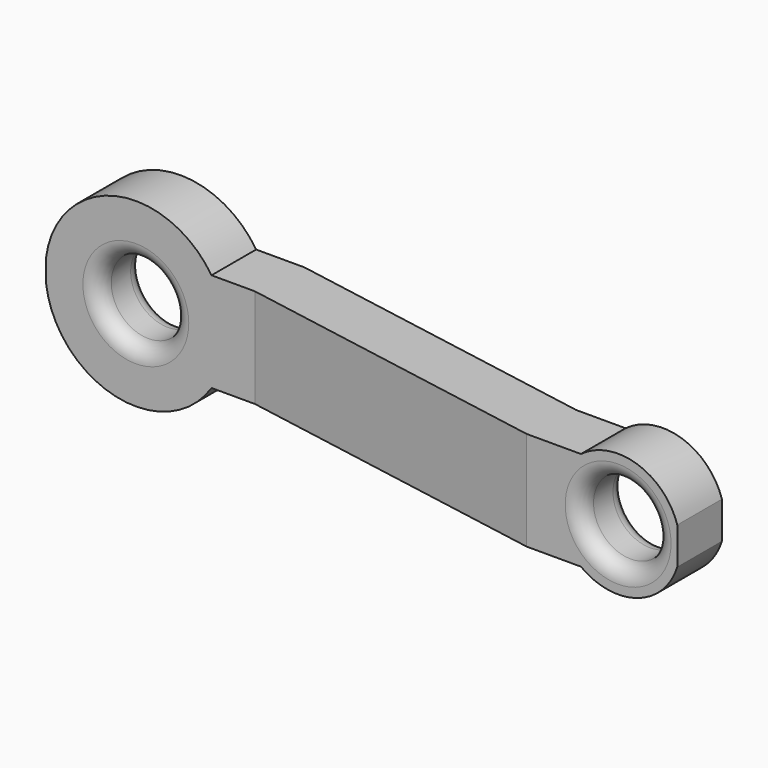
from build123d import *

# Parameters (mm, degrees)
F0_R     = 6
F1_DEPTH = 25
F3_DEPTH = 317.5
F4_R     = 2.54


with BuildPart() as f1:
    # F0 (on Front) → F1 (new body)
    with BuildSketch(Plane.XZ):
        with BuildLine():
            ThreePointArc((12.2088000741, -8), (13.9867667719, -4.1743448012), (14.59639679, 0))
            ThreePointArc((14.59639679, 0), (13.9867667719, 4.1743448012), (12.2088000741, 8))
            ThreePointArc((12.2088000741, 8), (-14.59639679, 0), (12.2088000741, -8))
        make_face()
        Circle(F0_R, mode=Mode.SUBTRACT)
        with BuildLine():
            ThreePointArc((12.2088000741, 8), (13.9867667719, 4.1743448012), (14.59639679, 0))
            ThreePointArc((14.59639679, 0), (13.9867667719, -4.1743448012), (12.2088000741, -8))
            Line((12.2088000741, -8), (79, -8))
            ThreePointArc((79, -8), (75, 0), (79, 8))
            Line((79, 8), (12.2088000741, 8))
        make_face()
        with BuildLine():
            ThreePointArc((95, 0), (89.472135955, 8.94427191), (79, 8))
            ThreePointArc((79, 8), (75, 0), (79, -8))
            ThreePointArc((79, -8), (89.472135955, -8.94427191), (95, 0))
        make_face()
        with Locations((85, 0)):
            Circle(F0_R, mode=Mode.SUBTRACT)
    extrude(amount=F1_DEPTH)

    # F2 (on Top) → F3 (intersect, symmetric)
    with BuildSketch(Plane.XY):
        Polygon((20, 0), (-14.4787151366, 0), (-14.4787151366, -9), (19.2126020283, -9), (70.2541384048, -18), (94.5431698973, -18), (94.5431698973, -9), (71.0415363766, -9), align=None)
    extrude(amount=F3_DEPTH, both=True, mode=Mode.INTERSECT)

    # F4
    f4_edges = [f1.edges().sort_by_distance(p)[0] for p in [
        (-6, -9, 0),
        (79, -18, 0),
        (-6, 0, 0),
        (79, -9, 0),
    ]]
    fillet(f4_edges, radius=F4_R)


solid = f1.part
